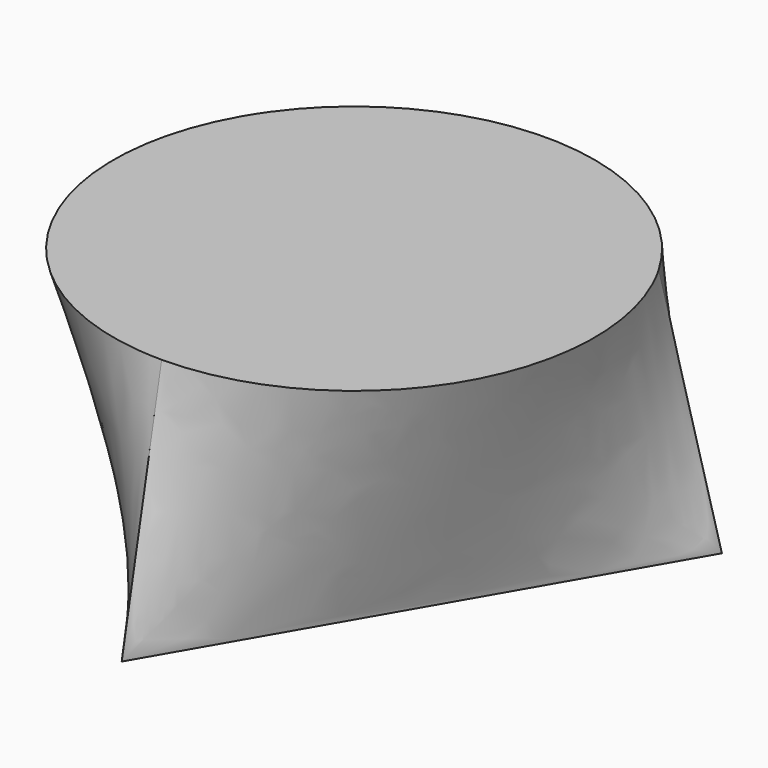
from build123d import *


# Not quite as in the source:
# - the arcs of a loft's sections are written as splines that run evenly, so that the points pair up as in the source's solid


with BuildPart() as f3:
    # F0 (on Top) → F3 section 0
    with BuildSketch(Plane.XY):
        Polygon((52.079182435, 30.067929998), (-52.079182435, 30.067929998), (0, -60.1358599961), align=None)
    # F2 (on offset) → F3 section 1
    with BuildSketch(Plane.XY.offset(50.8)):
        with BuildLine():
            add(Edge.make_bspline(
                [(43.1219648235, 24.8964779988), (41.673546446, 27.4052122192), (40.0056680218, 29.7871894663), (36.2815664752, 34.2254008636), (34.2254008636, 36.2815664752), (29.7871894663, 40.0056680218), (27.4052122192, 41.673546446), (22.3877437785, 44.5703832009), (19.7523300691, 45.799296796), (14.3080578248, 47.7808498402), (11.499283365, 48.5334586884), (5.7936287742, 49.5395195354), (2.8968367549, 49.7929559976), (-2.8968367549, 49.7929559976), (-5.7936287742, 49.5395195354), (-11.499283365, 48.5334586884), (-14.3080578248, 47.7808498402), (-19.7523300691, 45.799296796), (-22.3877437785, 44.5703832009), (-27.4052122192, 41.673546446), (-29.7871894663, 40.0056680218), (-34.2254008636, 36.2815664752), (-36.2815664752, 34.2254008636), (-40.0056680218, 29.7871894663), (-41.673546446, 27.4052122192), (-43.1219648235, 24.8964779988)],
                knots=[0, 0, 0, 0, 0.0833333333, 0.0833333333, 0.1666666667, 0.1666666667, 0.25, 0.25, 0.3333333333, 0.3333333333, 0.4166666667, 0.4166666667, 0.5, 0.5, 0.5833333333, 0.5833333333, 0.6666666667, 0.6666666667, 0.75, 0.75, 0.8333333333, 0.8333333333, 0.9166666667, 0.9166666667, 1, 1, 1, 1], degree=3))
            add(Edge.make_bspline(
                [(-43.1219648235, 24.8964779988), (-44.5703832009, 22.3877437785), (-45.799296796, 19.7523300691), (-47.7808498402, 14.3080578248), (-48.5334586884, 11.499283365), (-49.5395195354, 5.7936287742), (-49.7929559976, 2.8968367549), (-49.7929559976, -2.8968367549), (-49.5395195354, -5.7936287742), (-48.5334586884, -11.499283365), (-47.7808498402, -14.3080578248), (-45.799296796, -19.7523300691), (-44.5703832009, -22.3877437785), (-41.673546446, -27.4052122192), (-40.0056680218, -29.7871894663), (-36.2815664752, -34.2254008636), (-34.2254008636, -36.2815664752), (-29.7871894663, -40.0056680218), (-27.4052122192, -41.673546446), (-22.3877437785, -44.5703832009), (-19.7523300691, -45.799296796), (-14.3080578248, -47.7808498402), (-11.499283365, -48.5334586884), (-5.7936287742, -49.5395195354), (-2.8968367549, -49.7929559976), (0, -49.7929559976)],
                knots=[0, 0, 0, 0, 0.0833333333, 0.0833333333, 0.1666666667, 0.1666666667, 0.25, 0.25, 0.3333333333, 0.3333333333, 0.4166666667, 0.4166666667, 0.5, 0.5, 0.5833333333, 0.5833333333, 0.6666666667, 0.6666666667, 0.75, 0.75, 0.8333333333, 0.8333333333, 0.9166666667, 0.9166666667, 1, 1, 1, 1], degree=3))
            add(Edge.make_bspline(
                [(0, -49.7929559976), (2.8968367549, -49.7929559976), (5.7936287742, -49.5395195354), (11.499283365, -48.5334586884), (14.3080578248, -47.7808498402), (19.7523300691, -45.799296796), (22.3877437785, -44.5703832009), (27.4052122192, -41.673546446), (29.7871894663, -40.0056680218), (34.2254008636, -36.2815664752), (36.2815664752, -34.2254008636), (40.0056680218, -29.7871894663), (41.673546446, -27.4052122192), (44.5703832009, -22.3877437785), (45.799296796, -19.7523300691), (47.7808498402, -14.3080578248), (48.5334586884, -11.499283365), (49.5395195354, -5.7936287742), (49.7929559976, -2.8968367549), (49.7929559976, 2.8968367549), (49.5395195354, 5.7936287742), (48.5334586884, 11.499283365), (47.7808498402, 14.3080578248), (45.799296796, 19.7523300691), (44.5703832009, 22.3877437785), (43.1219648235, 24.8964779988)],
                knots=[0, 0, 0, 0, 0.0833333333, 0.0833333333, 0.1666666667, 0.1666666667, 0.25, 0.25, 0.3333333333, 0.3333333333, 0.4166666667, 0.4166666667, 0.5, 0.5, 0.5833333333, 0.5833333333, 0.6666666667, 0.6666666667, 0.75, 0.75, 0.8333333333, 0.8333333333, 0.9166666667, 0.9166666667, 1, 1, 1, 1], degree=3))
        make_face()
    loft(ruled=True)


solid = f3.part
